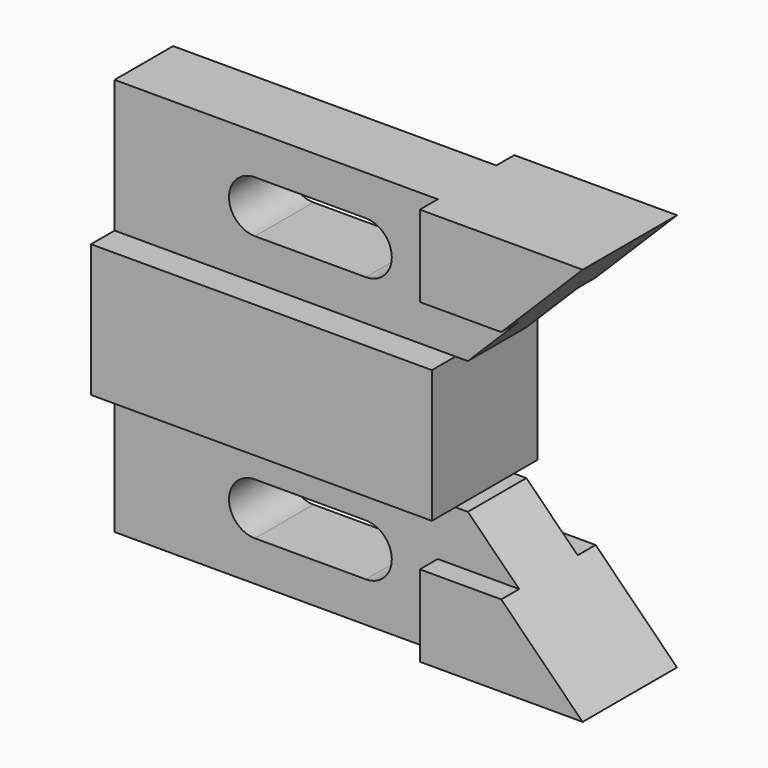
from build123d import *

# Parameters (mm, degrees)
F0_W     = 73.406
F0_H     = 28.575
F2_DEPTH = 14.224
F4_DEPTH = 7.874
F5_DEPTH = 12.7


# Not quite as in the source:
# - a pattern or mirror of a feature is missing from the dataset's text; its kind, count and spacing are read off the source's solid
# - a feature names something its author has since deleted; it is built from what else it names


with BuildPart() as f2:
    # F0 (on Front) → F2 (new body, symmetric)
    with BuildSketch(Plane.XZ):
        Rectangle(F0_W, F0_H)
    extrude(amount=F2_DEPTH, both=True)

    # F3 (on Front) → F4 (join, symmetric)
    with BuildSketch(Plane.XZ):
        Polygon((-36.703, -14.2875), (-36.703, -42.8625), (67.945, -42.8625), (39.37, -14.2875), align=None)
        with BuildLine():
            Line((-6.477, -23.0505), (17.399, -23.0505))
            ThreePointArc((17.399, -23.0505), (21.3503126933, -24.6871873067), (22.987, -28.6385))
            ThreePointArc((22.987, -28.6385), (21.3503126933, -32.5898126933), (17.399, -34.2265))
            Line((17.399, -34.2265), (-6.477, -34.2265))
            ThreePointArc((-6.477, -34.2265), (-12.065, -28.6385), (-6.477, -23.0505))
        make_face(mode=Mode.SUBTRACT)
        Polygon((-36.703, 14.2875), (36.703, 14.2875), (39.37, 14.2875), (50.419, 25.3365), (32.893, 25.3365), (32.893, 42.8625), (-36.703, 42.8625), align=None)
        with BuildLine():
            ThreePointArc((-6.477, 23.0505), (-12.065, 28.6385), (-6.477, 34.2265))
            Line((-6.477, 34.2265), (17.399, 34.2265))
            ThreePointArc((17.399, 34.2265), (21.3503126933, 32.5898126933), (22.987, 28.6385))
            ThreePointArc((22.987, 28.6385), (21.3503126933, 24.6871873067), (17.399, 23.0505))
            Line((17.399, 23.0505), (-6.477, 23.0505))
        make_face(mode=Mode.SUBTRACT)
        Polygon((32.893, 25.3365), (50.419, 25.3365), (67.945, 42.8625), (32.893, 42.8625), align=None)
    extrude(amount=F4_DEPTH, both=True)

    # F3 (on Front) → F5 (join, symmetric)
    with BuildSketch(Plane.XZ):
        Polygon((32.893, 25.3365), (50.419, 25.3365), (67.945, 42.8625), (32.893, 42.8625), align=None)
    f5 = extrude(amount=F5_DEPTH, both=True)

    # F5_copies: F5 across plane
    add(f5.mirror(Plane(origin=(0, 0, 0), x_dir=(-1, 0, 0), z_dir=(0, 0, -1))))


solid = f2.part
